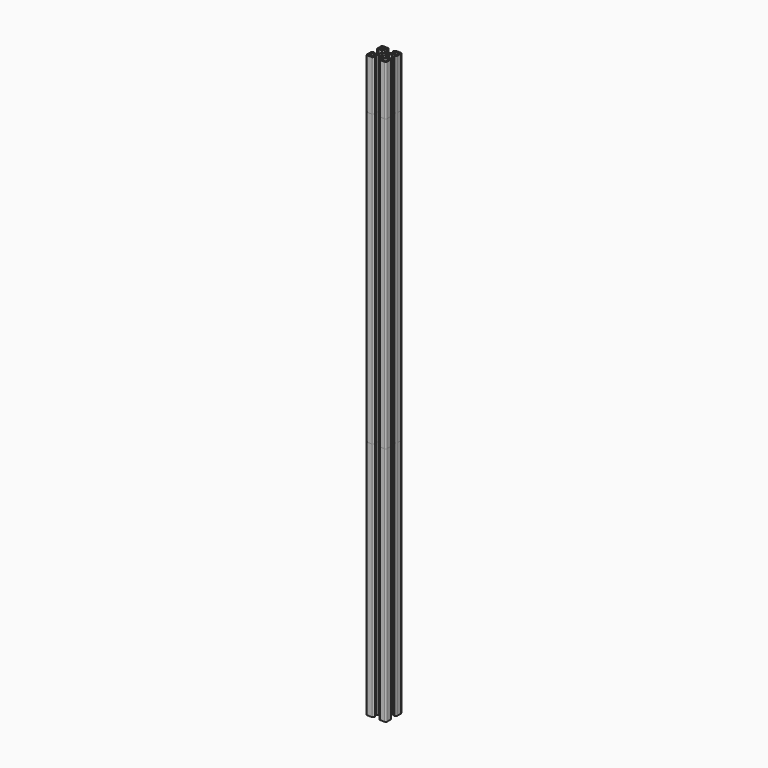
from build123d import *

# Parameters (mm, degrees)
F0_R     = 2.1
F1_DEPTH = 340
F2_DEPTH = 240
F3_DEPTH = 290


# Not quite as in the source:
# - ends of sketch curves that miss each other by under 0.0002 mm in the source are joined


with BuildPart() as f1:
    # F0 (on Top) → F1 (new body)
    with BuildSketch(Plane.XY):
        with BuildLine():
            ThreePointArc((-9.7686134352, -3.6910416547), (-9.9398646382, -3.9473364469), (-10.0000000781, -4.2496570118))
            Line((-10.0000000781, -4.2496570118), (-10.0000000781, -8.5808970118))
            ThreePointArc((-10.0000000781, -8.5808970118), (-9.5692783777, -9.55712574), (-8.5985020649, -9.9999998067))
            Line((-8.5985020649, -9.9999998067), (-4.0428310781, -10.0000000118))
            ThreePointArc((-4.0428310781, -10.0000000118), (-3.7366840055, -9.9391035025), (-3.4771451531, -9.7656849367))
            Line((-3.4771451531, -9.7656849367), (-2.3732230781, -8.6617630118))
            ThreePointArc((-2.3732230781, -8.6617630118), (-2.3190301949, -8.3893151537), (-2.5500000781, -8.2349860118))
            Line((-2.5500000781, -8.2349860118), (-3.6000000781, -8.2349860118))
            Line((-3.6000000781, -8.2349860118), (-3.6000000781, -5.0349860118))
            Line((-3.6000000781, -5.0349860118), (-2.0054060781, -3.4349860118))
            Line((-2.0054060781, -3.4349860118), (-0.3000000781, -3.4349860118))
            Line((-0.3000000781, -3.4349860118), (-7.81e-08, -3.1750330118))
            Line((-7.81e-08, -3.1750330118), (0.2999999219, -3.4349860118))
            Line((0.2999999219, -3.4349860118), (2.0054059219, -3.4349860118))
            Line((2.0054059219, -3.4349860118), (3.5999999219, -5.0349860118))
            Line((3.5999999219, -5.0349860118), (3.5999999219, -8.2349860118))
            Line((3.5999999219, -8.2349860118), (2.5499999219, -8.2349860118))
            ThreePointArc((2.5499999219, -8.2349860118), (2.3190299035, -8.3893154803), (2.3732237266, -8.6617632071))
            Line((2.3732237266, -8.6617632071), (3.4771459219, -9.7656850118))
            ThreePointArc((3.4771459219, -9.7656850118), (3.736684176, -9.9391036378), (4.0428309219, -10.0000000118))
            Line((4.0428309219, -10.0000000118), (8.5985019219, -10.0000000118))
            ThreePointArc((8.5985019219, -10.0000000118), (9.5692782397, -9.5571257216), (10.0000004186, -8.5808969857))
            Line((10.0000004186, -8.5808969857), (9.9999999219, -4.2496570118))
            ThreePointArc((9.9999999219, -4.2496570118), (9.9398646173, -3.9473367736), (9.7686137791, -3.6910421547))
            Line((9.7686137791, -3.6910421547), (8.4861509219, -2.4085790118))
            ThreePointArc((8.4861509219, -2.4085790118), (8.2729345349, -2.363330341), (8.1449896008, -2.5397919954))
            Line((8.1449896008, -2.5397919954), (8.1449899219, -3.6000000118))
            Line((8.1449899219, -3.6000000118), (5.0283829219, -3.6000000118))
            Line((5.0283829219, -3.6000000118), (3.3999999219, -1.9660960118))
            Line((3.3999999219, -1.9660960118), (3.3999999219, -0.3808970118))
            Line((3.3999999219, -0.3808970118), (3.0191029219, -1.18e-08))
            Line((3.0191029219, -1.18e-08), (3.3999999219, 0.3808969882))
            Line((3.3999999219, 0.3808969882), (3.3999999219, 1.9660959882))
            Line((3.3999999219, 1.9660959882), (5.0283829219, 3.5999999882))
            Line((5.0283829219, 3.5999999882), (8.1449899219, 3.5999999882))
            Line((8.1449899219, 3.5999999882), (8.1449899219, 2.5397919882))
            ThreePointArc((8.1449899219, 2.5397919882), (8.2729345349, 2.3633303174), (8.4861507782, 2.408579132))
            Line((8.4861507782, 2.408579132), (9.7686139219, 3.6910419882))
            ThreePointArc((9.7686139219, 3.6910419882), (9.9398646173, 3.94733675), (9.9999999219, 4.2496569882))
            Line((9.9999999219, 4.2496569882), (9.9999999219, 8.5808969882))
            ThreePointArc((9.9999999219, 8.5808969882), (9.5692782397, 9.557125698), (8.5985019087, 9.9999997831))
            Line((8.5985019087, 9.9999997831), (4.0428309219, 9.9999999882))
            ThreePointArc((4.0428309219, 9.9999999882), (3.7366845027, 9.9391037495), (3.477145997, 9.7656859132))
            Line((3.477145997, 9.7656859132), (2.3732229219, 8.6617629882))
            ThreePointArc((2.3732229219, 8.6617629882), (2.3190299035, 8.3893154568), (2.5499999219, 8.2349859882))
            Line((2.5499999219, 8.2349859882), (3.5999999219, 8.2349859882))
            Line((3.5999999219, 8.2349859882), (3.5999999219, 5.0349859882))
            Line((3.5999999219, 5.0349859882), (2.0054059219, 3.4349859882))
            Line((2.0054059219, 3.4349859882), (0.2999999219, 3.4349859882))
            Line((0.2999999219, 3.4349859882), (-7.81e-08, 3.1750329882))
            Line((-7.81e-08, 3.1750329882), (-0.3000000781, 3.4349859882))
            Line((-0.3000000781, 3.4349859882), (-2.0054060781, 3.4349859882))
            Line((-2.0054060781, 3.4349859882), (-3.6000000781, 5.0349859882))
            Line((-3.6000000781, 5.0349859882), (-3.6000000781, 8.2349859882))
            Line((-3.6000000781, 8.2349859882), (-2.5500000781, 8.2349859882))
            ThreePointArc((-2.5500000781, 8.2349859882), (-2.3190301949, 8.3893151301), (-2.3732233828, 8.6617626835))
            Line((-2.3732233828, 8.6617626835), (-3.4771460781, 9.7656849882))
            ThreePointArc((-3.4771460781, 9.7656849882), (-3.7366843322, 9.9391036142), (-4.0428310781, 9.9999999882))
            Line((-4.0428310781, 9.9999999882), (-8.5985020781, 9.9999999882))
            ThreePointArc((-8.5985020781, 9.9999999882), (-9.5692783777, 9.5571257164), (-10.0000005721, 8.5808970139))
            Line((-10.0000005721, 8.5808970139), (-10.0000000781, 4.2496569882))
            ThreePointArc((-10.0000000781, 4.2496569882), (-9.9398646382, 3.9473364234), (-9.7686134352, 3.6910416311))
            Line((-9.7686134352, 3.6910416311), (-8.4861510781, 2.4085789882))
            ThreePointArc((-8.4861510781, 2.4085789882), (-8.2729343372, 2.3633304535), (-8.1449897544, 2.5397920228))
            Line((-8.1449897544, 2.5397920228), (-8.1449900781, 3.5999999882))
            Line((-8.1449900781, 3.5999999882), (-5.0283830781, 3.5999999882))
            Line((-5.0283830781, 3.5999999882), (-3.4000000781, 1.9660959882))
            Line((-3.4000000781, 1.9660959882), (-3.4000000781, 0.3808969882))
            Line((-3.4000000781, 0.3808969882), (-3.0191030781, -1.18e-08))
            Line((-3.0191030781, -1.18e-08), (-3.4000000781, -0.3808970118))
            Line((-3.4000000781, -0.3808970118), (-3.4000000781, -1.9660960118))
            Line((-3.4000000781, -1.9660960118), (-5.0283830781, -3.6000000118))
            Line((-5.0283830781, -3.6000000118), (-8.1449900781, -3.6000000118))
            Line((-8.1449900781, -3.6000000118), (-8.1449900781, -2.5397920118))
            ThreePointArc((-8.1449900781, -2.5397920118), (-8.2729343372, -2.3633304771), (-8.4861504343, -2.4085786556))
            Line((-8.4861504343, -2.4085786556), (-9.7686134352, -3.6910416547))
        make_face()
        with BuildLine():
            Line((-8.3887380781, -4.8000000118), (-5.3887380781, -4.8000000118))
            ThreePointArc((-5.3887380781, -4.8000000118), (-4.9405858182, -4.9345893802), (-4.7999996469, -5.3808969072))
            Line((-4.7999996469, -5.3808969072), (-4.8000000781, -8.3808970118))
            ThreePointArc((-4.8000000781, -8.3808970118), (-5.0082631765, -8.7203831526), (-5.3985012393, -8.7999997745))
            Line((-5.3985012393, -8.7999997745), (-8.3985020781, -8.8000000118))
            ThreePointArc((-8.3985020781, -8.8000000118), (-8.6662843252, -8.6546658791), (-8.8000004374, -8.3808970642))
            Line((-8.8000004374, -8.3808970642), (-8.8000000781, -5.3808970118))
            ThreePointArc((-8.8000000781, -5.3808970118), (-8.7157976891, -5.0044798887), (-8.3887380781, -4.8000000118))
        make_face(mode=Mode.SUBTRACT)
        with Locations((-7.81e-08, -1.18e-08)):
            Circle(F0_R, mode=Mode.SUBTRACT)
        with BuildLine():
            ThreePointArc((8.3887379109, -4.800000079), (8.7157974824, -5.0044798173), (8.8000002705, -5.380896896))
            Line((8.8000002705, -5.380896896), (8.8000009219, -8.3808970118))
            ThreePointArc((8.8000009219, -8.3808970118), (8.6662842189, -8.654665827), (8.3985019428, -8.8000001216))
            Line((8.3985019428, -8.8000001216), (5.3985019219, -8.8000000118))
            ThreePointArc((5.3985019219, -8.8000000118), (5.0082634784, -8.7203834734), (4.7999996354, -8.3808970523))
            Line((4.7999996354, -8.3808970523), (4.7999999219, -5.3808970118))
            ThreePointArc((4.7999999219, -5.3808970118), (4.9405855977, -4.9345894436), (5.3887379814, -4.7999997112))
            Line((5.3887379814, -4.7999997112), (8.3887379109, -4.800000079))
        make_face(mode=Mode.SUBTRACT)
        with BuildLine():
            ThreePointArc((-8.388738067, 4.8000000554), (-8.7157976891, 5.0044798651), (-8.800000396, 5.3808970447))
            Line((-8.800000396, 5.3808970447), (-8.8000000781, 8.3808969882))
            ThreePointArc((-8.8000000781, 8.3808969882), (-8.6662843252, 8.6546658555), (-8.3985020989, 8.800000098))
            Line((-8.3985020989, 8.800000098), (-5.3985020781, 8.7999999882))
            ThreePointArc((-5.3985020781, 8.7999999882), (-5.0082630918, 8.7203830697), (-4.7999997719, 8.38089689))
            Line((-4.7999997719, 8.38089689), (-4.8000000781, 5.3808969882))
            ThreePointArc((-4.8000000781, 5.3808969882), (-4.9405858182, 4.9345893566), (-5.3887381375, 4.7999996876))
            Line((-5.3887381375, 4.7999996876), (-8.388738067, 4.8000000554))
        make_face(mode=Mode.SUBTRACT)
        with BuildLine():
            Line((8.3887379219, 4.7999999882), (5.3887379219, 4.7999999882))
            ThreePointArc((5.3887379219, 4.7999999882), (4.9405855977, 4.9345894201), (4.7999995234, 5.3808970615))
            Line((4.7999995234, 5.3808970615), (4.7999999219, 8.3808969882))
            ThreePointArc((4.7999999219, 8.3808969882), (5.0082633937, 8.7203833905), (5.398501838, 8.7999995913))
            Line((5.398501838, 8.7999995913), (8.3985019219, 8.7999999882))
            ThreePointArc((8.3985019219, 8.7999999882), (8.6662842189, 8.6546658035), (8.8000003021, 8.3808968979))
            Line((8.8000003021, 8.3808968979), (8.7999999219, 5.3808969882))
            ThreePointArc((8.7999999219, 5.3808969882), (8.7157974824, 5.0044797937), (8.3887379219, 4.7999999882))
        make_face(mode=Mode.SUBTRACT)
    extrude(amount=F1_DEPTH)


with BuildPart() as f2:
    # F0 (on Top) → F2 (new body)
    with BuildSketch(Plane.XY):
        with BuildLine():
            ThreePointArc((-9.7686134352, -3.6910416547), (-9.9398646382, -3.9473364469), (-10.0000000781, -4.2496570118))
            Line((-10.0000000781, -4.2496570118), (-10.0000000781, -8.5808970118))
            ThreePointArc((-10.0000000781, -8.5808970118), (-9.5692783777, -9.55712574), (-8.5985020649, -9.9999998067))
            Line((-8.5985020649, -9.9999998067), (-4.0428310781, -10.0000000118))
            ThreePointArc((-4.0428310781, -10.0000000118), (-3.7366840055, -9.9391035025), (-3.4771451531, -9.7656849367))
            Line((-3.4771451531, -9.7656849367), (-2.3732230781, -8.6617630118))
            ThreePointArc((-2.3732230781, -8.6617630118), (-2.3190301949, -8.3893151537), (-2.5500000781, -8.2349860118))
            Line((-2.5500000781, -8.2349860118), (-3.6000000781, -8.2349860118))
            Line((-3.6000000781, -8.2349860118), (-3.6000000781, -5.0349860118))
            Line((-3.6000000781, -5.0349860118), (-2.0054060781, -3.4349860118))
            Line((-2.0054060781, -3.4349860118), (-0.3000000781, -3.4349860118))
            Line((-0.3000000781, -3.4349860118), (-7.81e-08, -3.1750330118))
            Line((-7.81e-08, -3.1750330118), (0.2999999219, -3.4349860118))
            Line((0.2999999219, -3.4349860118), (2.0054059219, -3.4349860118))
            Line((2.0054059219, -3.4349860118), (3.5999999219, -5.0349860118))
            Line((3.5999999219, -5.0349860118), (3.5999999219, -8.2349860118))
            Line((3.5999999219, -8.2349860118), (2.5499999219, -8.2349860118))
            ThreePointArc((2.5499999219, -8.2349860118), (2.3190299035, -8.3893154803), (2.3732237266, -8.6617632071))
            Line((2.3732237266, -8.6617632071), (3.4771459219, -9.7656850118))
            ThreePointArc((3.4771459219, -9.7656850118), (3.736684176, -9.9391036378), (4.0428309219, -10.0000000118))
            Line((4.0428309219, -10.0000000118), (8.5985019219, -10.0000000118))
            ThreePointArc((8.5985019219, -10.0000000118), (9.5692782397, -9.5571257216), (10.0000004186, -8.5808969857))
            Line((10.0000004186, -8.5808969857), (9.9999999219, -4.2496570118))
            ThreePointArc((9.9999999219, -4.2496570118), (9.9398646173, -3.9473367736), (9.7686137791, -3.6910421547))
            Line((9.7686137791, -3.6910421547), (8.4861509219, -2.4085790118))
            ThreePointArc((8.4861509219, -2.4085790118), (8.2729345349, -2.363330341), (8.1449896008, -2.5397919954))
            Line((8.1449896008, -2.5397919954), (8.1449899219, -3.6000000118))
            Line((8.1449899219, -3.6000000118), (5.0283829219, -3.6000000118))
            Line((5.0283829219, -3.6000000118), (3.3999999219, -1.9660960118))
            Line((3.3999999219, -1.9660960118), (3.3999999219, -0.3808970118))
            Line((3.3999999219, -0.3808970118), (3.0191029219, -1.18e-08))
            Line((3.0191029219, -1.18e-08), (3.3999999219, 0.3808969882))
            Line((3.3999999219, 0.3808969882), (3.3999999219, 1.9660959882))
            Line((3.3999999219, 1.9660959882), (5.0283829219, 3.5999999882))
            Line((5.0283829219, 3.5999999882), (8.1449899219, 3.5999999882))
            Line((8.1449899219, 3.5999999882), (8.1449899219, 2.5397919882))
            ThreePointArc((8.1449899219, 2.5397919882), (8.2729345349, 2.3633303174), (8.4861507782, 2.408579132))
            Line((8.4861507782, 2.408579132), (9.7686139219, 3.6910419882))
            ThreePointArc((9.7686139219, 3.6910419882), (9.9398646173, 3.94733675), (9.9999999219, 4.2496569882))
            Line((9.9999999219, 4.2496569882), (9.9999999219, 8.5808969882))
            ThreePointArc((9.9999999219, 8.5808969882), (9.5692782397, 9.557125698), (8.5985019087, 9.9999997831))
            Line((8.5985019087, 9.9999997831), (4.0428309219, 9.9999999882))
            ThreePointArc((4.0428309219, 9.9999999882), (3.7366845027, 9.9391037495), (3.477145997, 9.7656859132))
            Line((3.477145997, 9.7656859132), (2.3732229219, 8.6617629882))
            ThreePointArc((2.3732229219, 8.6617629882), (2.3190299035, 8.3893154568), (2.5499999219, 8.2349859882))
            Line((2.5499999219, 8.2349859882), (3.5999999219, 8.2349859882))
            Line((3.5999999219, 8.2349859882), (3.5999999219, 5.0349859882))
            Line((3.5999999219, 5.0349859882), (2.0054059219, 3.4349859882))
            Line((2.0054059219, 3.4349859882), (0.2999999219, 3.4349859882))
            Line((0.2999999219, 3.4349859882), (-7.81e-08, 3.1750329882))
            Line((-7.81e-08, 3.1750329882), (-0.3000000781, 3.4349859882))
            Line((-0.3000000781, 3.4349859882), (-2.0054060781, 3.4349859882))
            Line((-2.0054060781, 3.4349859882), (-3.6000000781, 5.0349859882))
            Line((-3.6000000781, 5.0349859882), (-3.6000000781, 8.2349859882))
            Line((-3.6000000781, 8.2349859882), (-2.5500000781, 8.2349859882))
            ThreePointArc((-2.5500000781, 8.2349859882), (-2.3190301949, 8.3893151301), (-2.3732233828, 8.6617626835))
            Line((-2.3732233828, 8.6617626835), (-3.4771460781, 9.7656849882))
            ThreePointArc((-3.4771460781, 9.7656849882), (-3.7366843322, 9.9391036142), (-4.0428310781, 9.9999999882))
            Line((-4.0428310781, 9.9999999882), (-8.5985020781, 9.9999999882))
            ThreePointArc((-8.5985020781, 9.9999999882), (-9.5692783777, 9.5571257164), (-10.0000005721, 8.5808970139))
            Line((-10.0000005721, 8.5808970139), (-10.0000000781, 4.2496569882))
            ThreePointArc((-10.0000000781, 4.2496569882), (-9.9398646382, 3.9473364234), (-9.7686134352, 3.6910416311))
            Line((-9.7686134352, 3.6910416311), (-8.4861510781, 2.4085789882))
            ThreePointArc((-8.4861510781, 2.4085789882), (-8.2729343372, 2.3633304535), (-8.1449897544, 2.5397920228))
            Line((-8.1449897544, 2.5397920228), (-8.1449900781, 3.5999999882))
            Line((-8.1449900781, 3.5999999882), (-5.0283830781, 3.5999999882))
            Line((-5.0283830781, 3.5999999882), (-3.4000000781, 1.9660959882))
            Line((-3.4000000781, 1.9660959882), (-3.4000000781, 0.3808969882))
            Line((-3.4000000781, 0.3808969882), (-3.0191030781, -1.18e-08))
            Line((-3.0191030781, -1.18e-08), (-3.4000000781, -0.3808970118))
            Line((-3.4000000781, -0.3808970118), (-3.4000000781, -1.9660960118))
            Line((-3.4000000781, -1.9660960118), (-5.0283830781, -3.6000000118))
            Line((-5.0283830781, -3.6000000118), (-8.1449900781, -3.6000000118))
            Line((-8.1449900781, -3.6000000118), (-8.1449900781, -2.5397920118))
            ThreePointArc((-8.1449900781, -2.5397920118), (-8.2729343372, -2.3633304771), (-8.4861504343, -2.4085786556))
            Line((-8.4861504343, -2.4085786556), (-9.7686134352, -3.6910416547))
        make_face()
        with BuildLine():
            Line((-8.3887380781, -4.8000000118), (-5.3887380781, -4.8000000118))
            ThreePointArc((-5.3887380781, -4.8000000118), (-4.9405858182, -4.9345893802), (-4.7999996469, -5.3808969072))
            Line((-4.7999996469, -5.3808969072), (-4.8000000781, -8.3808970118))
            ThreePointArc((-4.8000000781, -8.3808970118), (-5.0082631765, -8.7203831526), (-5.3985012393, -8.7999997745))
            Line((-5.3985012393, -8.7999997745), (-8.3985020781, -8.8000000118))
            ThreePointArc((-8.3985020781, -8.8000000118), (-8.6662843252, -8.6546658791), (-8.8000004374, -8.3808970642))
            Line((-8.8000004374, -8.3808970642), (-8.8000000781, -5.3808970118))
            ThreePointArc((-8.8000000781, -5.3808970118), (-8.7157976891, -5.0044798887), (-8.3887380781, -4.8000000118))
        make_face(mode=Mode.SUBTRACT)
        with Locations((-7.81e-08, -1.18e-08)):
            Circle(F0_R, mode=Mode.SUBTRACT)
        with BuildLine():
            ThreePointArc((8.3887379109, -4.800000079), (8.7157974824, -5.0044798173), (8.8000002705, -5.380896896))
            Line((8.8000002705, -5.380896896), (8.8000009219, -8.3808970118))
            ThreePointArc((8.8000009219, -8.3808970118), (8.6662842189, -8.654665827), (8.3985019428, -8.8000001216))
            Line((8.3985019428, -8.8000001216), (5.3985019219, -8.8000000118))
            ThreePointArc((5.3985019219, -8.8000000118), (5.0082634784, -8.7203834734), (4.7999996354, -8.3808970523))
            Line((4.7999996354, -8.3808970523), (4.7999999219, -5.3808970118))
            ThreePointArc((4.7999999219, -5.3808970118), (4.9405855977, -4.9345894436), (5.3887379814, -4.7999997112))
            Line((5.3887379814, -4.7999997112), (8.3887379109, -4.800000079))
        make_face(mode=Mode.SUBTRACT)
        with BuildLine():
            ThreePointArc((-8.388738067, 4.8000000554), (-8.7157976891, 5.0044798651), (-8.800000396, 5.3808970447))
            Line((-8.800000396, 5.3808970447), (-8.8000000781, 8.3808969882))
            ThreePointArc((-8.8000000781, 8.3808969882), (-8.6662843252, 8.6546658555), (-8.3985020989, 8.800000098))
            Line((-8.3985020989, 8.800000098), (-5.3985020781, 8.7999999882))
            ThreePointArc((-5.3985020781, 8.7999999882), (-5.0082630918, 8.7203830697), (-4.7999997719, 8.38089689))
            Line((-4.7999997719, 8.38089689), (-4.8000000781, 5.3808969882))
            ThreePointArc((-4.8000000781, 5.3808969882), (-4.9405858182, 4.9345893566), (-5.3887381375, 4.7999996876))
            Line((-5.3887381375, 4.7999996876), (-8.388738067, 4.8000000554))
        make_face(mode=Mode.SUBTRACT)
        with BuildLine():
            Line((8.3887379219, 4.7999999882), (5.3887379219, 4.7999999882))
            ThreePointArc((5.3887379219, 4.7999999882), (4.9405855977, 4.9345894201), (4.7999995234, 5.3808970615))
            Line((4.7999995234, 5.3808970615), (4.7999999219, 8.3808969882))
            ThreePointArc((4.7999999219, 8.3808969882), (5.0082633937, 8.7203833905), (5.398501838, 8.7999995913))
            Line((5.398501838, 8.7999995913), (8.3985019219, 8.7999999882))
            ThreePointArc((8.3985019219, 8.7999999882), (8.6662842189, 8.6546658035), (8.8000003021, 8.3808968979))
            Line((8.8000003021, 8.3808968979), (8.7999999219, 5.3808969882))
            ThreePointArc((8.7999999219, 5.3808969882), (8.7157974824, 5.0044797937), (8.3887379219, 4.7999999882))
        make_face(mode=Mode.SUBTRACT)
    extrude(amount=-F2_DEPTH)


with BuildPart() as f3:
    # F0 (on Top) → F3 (new body)
    with BuildSketch(Plane.XY):
        with BuildLine():
            ThreePointArc((-9.7686134352, -3.6910416547), (-9.9398646382, -3.9473364469), (-10.0000000781, -4.2496570118))
            Line((-10.0000000781, -4.2496570118), (-10.0000000781, -8.5808970118))
            ThreePointArc((-10.0000000781, -8.5808970118), (-9.5692783777, -9.55712574), (-8.5985020649, -9.9999998067))
            Line((-8.5985020649, -9.9999998067), (-4.0428310781, -10.0000000118))
            ThreePointArc((-4.0428310781, -10.0000000118), (-3.7366840055, -9.9391035025), (-3.4771451531, -9.7656849367))
            Line((-3.4771451531, -9.7656849367), (-2.3732230781, -8.6617630118))
            ThreePointArc((-2.3732230781, -8.6617630118), (-2.3190301949, -8.3893151537), (-2.5500000781, -8.2349860118))
            Line((-2.5500000781, -8.2349860118), (-3.6000000781, -8.2349860118))
            Line((-3.6000000781, -8.2349860118), (-3.6000000781, -5.0349860118))
            Line((-3.6000000781, -5.0349860118), (-2.0054060781, -3.4349860118))
            Line((-2.0054060781, -3.4349860118), (-0.3000000781, -3.4349860118))
            Line((-0.3000000781, -3.4349860118), (-7.81e-08, -3.1750330118))
            Line((-7.81e-08, -3.1750330118), (0.2999999219, -3.4349860118))
            Line((0.2999999219, -3.4349860118), (2.0054059219, -3.4349860118))
            Line((2.0054059219, -3.4349860118), (3.5999999219, -5.0349860118))
            Line((3.5999999219, -5.0349860118), (3.5999999219, -8.2349860118))
            Line((3.5999999219, -8.2349860118), (2.5499999219, -8.2349860118))
            ThreePointArc((2.5499999219, -8.2349860118), (2.3190299035, -8.3893154803), (2.3732237266, -8.6617632071))
            Line((2.3732237266, -8.6617632071), (3.4771459219, -9.7656850118))
            ThreePointArc((3.4771459219, -9.7656850118), (3.736684176, -9.9391036378), (4.0428309219, -10.0000000118))
            Line((4.0428309219, -10.0000000118), (8.5985019219, -10.0000000118))
            ThreePointArc((8.5985019219, -10.0000000118), (9.5692782397, -9.5571257216), (10.0000004186, -8.5808969857))
            Line((10.0000004186, -8.5808969857), (9.9999999219, -4.2496570118))
            ThreePointArc((9.9999999219, -4.2496570118), (9.9398646173, -3.9473367736), (9.7686137791, -3.6910421547))
            Line((9.7686137791, -3.6910421547), (8.4861509219, -2.4085790118))
            ThreePointArc((8.4861509219, -2.4085790118), (8.2729345349, -2.363330341), (8.1449896008, -2.5397919954))
            Line((8.1449896008, -2.5397919954), (8.1449899219, -3.6000000118))
            Line((8.1449899219, -3.6000000118), (5.0283829219, -3.6000000118))
            Line((5.0283829219, -3.6000000118), (3.3999999219, -1.9660960118))
            Line((3.3999999219, -1.9660960118), (3.3999999219, -0.3808970118))
            Line((3.3999999219, -0.3808970118), (3.0191029219, -1.18e-08))
            Line((3.0191029219, -1.18e-08), (3.3999999219, 0.3808969882))
            Line((3.3999999219, 0.3808969882), (3.3999999219, 1.9660959882))
            Line((3.3999999219, 1.9660959882), (5.0283829219, 3.5999999882))
            Line((5.0283829219, 3.5999999882), (8.1449899219, 3.5999999882))
            Line((8.1449899219, 3.5999999882), (8.1449899219, 2.5397919882))
            ThreePointArc((8.1449899219, 2.5397919882), (8.2729345349, 2.3633303174), (8.4861507782, 2.408579132))
            Line((8.4861507782, 2.408579132), (9.7686139219, 3.6910419882))
            ThreePointArc((9.7686139219, 3.6910419882), (9.9398646173, 3.94733675), (9.9999999219, 4.2496569882))
            Line((9.9999999219, 4.2496569882), (9.9999999219, 8.5808969882))
            ThreePointArc((9.9999999219, 8.5808969882), (9.5692782397, 9.557125698), (8.5985019087, 9.9999997831))
            Line((8.5985019087, 9.9999997831), (4.0428309219, 9.9999999882))
            ThreePointArc((4.0428309219, 9.9999999882), (3.7366845027, 9.9391037495), (3.477145997, 9.7656859132))
            Line((3.477145997, 9.7656859132), (2.3732229219, 8.6617629882))
            ThreePointArc((2.3732229219, 8.6617629882), (2.3190299035, 8.3893154568), (2.5499999219, 8.2349859882))
            Line((2.5499999219, 8.2349859882), (3.5999999219, 8.2349859882))
            Line((3.5999999219, 8.2349859882), (3.5999999219, 5.0349859882))
            Line((3.5999999219, 5.0349859882), (2.0054059219, 3.4349859882))
            Line((2.0054059219, 3.4349859882), (0.2999999219, 3.4349859882))
            Line((0.2999999219, 3.4349859882), (-7.81e-08, 3.1750329882))
            Line((-7.81e-08, 3.1750329882), (-0.3000000781, 3.4349859882))
            Line((-0.3000000781, 3.4349859882), (-2.0054060781, 3.4349859882))
            Line((-2.0054060781, 3.4349859882), (-3.6000000781, 5.0349859882))
            Line((-3.6000000781, 5.0349859882), (-3.6000000781, 8.2349859882))
            Line((-3.6000000781, 8.2349859882), (-2.5500000781, 8.2349859882))
            ThreePointArc((-2.5500000781, 8.2349859882), (-2.3190301949, 8.3893151301), (-2.3732233828, 8.6617626835))
            Line((-2.3732233828, 8.6617626835), (-3.4771460781, 9.7656849882))
            ThreePointArc((-3.4771460781, 9.7656849882), (-3.7366843322, 9.9391036142), (-4.0428310781, 9.9999999882))
            Line((-4.0428310781, 9.9999999882), (-8.5985020781, 9.9999999882))
            ThreePointArc((-8.5985020781, 9.9999999882), (-9.5692783777, 9.5571257164), (-10.0000005721, 8.5808970139))
            Line((-10.0000005721, 8.5808970139), (-10.0000000781, 4.2496569882))
            ThreePointArc((-10.0000000781, 4.2496569882), (-9.9398646382, 3.9473364234), (-9.7686134352, 3.6910416311))
            Line((-9.7686134352, 3.6910416311), (-8.4861510781, 2.4085789882))
            ThreePointArc((-8.4861510781, 2.4085789882), (-8.2729343372, 2.3633304535), (-8.1449897544, 2.5397920228))
            Line((-8.1449897544, 2.5397920228), (-8.1449900781, 3.5999999882))
            Line((-8.1449900781, 3.5999999882), (-5.0283830781, 3.5999999882))
            Line((-5.0283830781, 3.5999999882), (-3.4000000781, 1.9660959882))
            Line((-3.4000000781, 1.9660959882), (-3.4000000781, 0.3808969882))
            Line((-3.4000000781, 0.3808969882), (-3.0191030781, -1.18e-08))
            Line((-3.0191030781, -1.18e-08), (-3.4000000781, -0.3808970118))
            Line((-3.4000000781, -0.3808970118), (-3.4000000781, -1.9660960118))
            Line((-3.4000000781, -1.9660960118), (-5.0283830781, -3.6000000118))
            Line((-5.0283830781, -3.6000000118), (-8.1449900781, -3.6000000118))
            Line((-8.1449900781, -3.6000000118), (-8.1449900781, -2.5397920118))
            ThreePointArc((-8.1449900781, -2.5397920118), (-8.2729343372, -2.3633304771), (-8.4861504343, -2.4085786556))
            Line((-8.4861504343, -2.4085786556), (-9.7686134352, -3.6910416547))
        make_face()
        with BuildLine():
            Line((-8.3887380781, -4.8000000118), (-5.3887380781, -4.8000000118))
            ThreePointArc((-5.3887380781, -4.8000000118), (-4.9405858182, -4.9345893802), (-4.7999996469, -5.3808969072))
            Line((-4.7999996469, -5.3808969072), (-4.8000000781, -8.3808970118))
            ThreePointArc((-4.8000000781, -8.3808970118), (-5.0082631765, -8.7203831526), (-5.3985012393, -8.7999997745))
            Line((-5.3985012393, -8.7999997745), (-8.3985020781, -8.8000000118))
            ThreePointArc((-8.3985020781, -8.8000000118), (-8.6662843252, -8.6546658791), (-8.8000004374, -8.3808970642))
            Line((-8.8000004374, -8.3808970642), (-8.8000000781, -5.3808970118))
            ThreePointArc((-8.8000000781, -5.3808970118), (-8.7157976891, -5.0044798887), (-8.3887380781, -4.8000000118))
        make_face(mode=Mode.SUBTRACT)
        with Locations((-7.81e-08, -1.18e-08)):
            Circle(F0_R, mode=Mode.SUBTRACT)
        with BuildLine():
            ThreePointArc((8.3887379109, -4.800000079), (8.7157974824, -5.0044798173), (8.8000002705, -5.380896896))
            Line((8.8000002705, -5.380896896), (8.8000009219, -8.3808970118))
            ThreePointArc((8.8000009219, -8.3808970118), (8.6662842189, -8.654665827), (8.3985019428, -8.8000001216))
            Line((8.3985019428, -8.8000001216), (5.3985019219, -8.8000000118))
            ThreePointArc((5.3985019219, -8.8000000118), (5.0082634784, -8.7203834734), (4.7999996354, -8.3808970523))
            Line((4.7999996354, -8.3808970523), (4.7999999219, -5.3808970118))
            ThreePointArc((4.7999999219, -5.3808970118), (4.9405855977, -4.9345894436), (5.3887379814, -4.7999997112))
            Line((5.3887379814, -4.7999997112), (8.3887379109, -4.800000079))
        make_face(mode=Mode.SUBTRACT)
        with BuildLine():
            ThreePointArc((-8.388738067, 4.8000000554), (-8.7157976891, 5.0044798651), (-8.800000396, 5.3808970447))
            Line((-8.800000396, 5.3808970447), (-8.8000000781, 8.3808969882))
            ThreePointArc((-8.8000000781, 8.3808969882), (-8.6662843252, 8.6546658555), (-8.3985020989, 8.800000098))
            Line((-8.3985020989, 8.800000098), (-5.3985020781, 8.7999999882))
            ThreePointArc((-5.3985020781, 8.7999999882), (-5.0082630918, 8.7203830697), (-4.7999997719, 8.38089689))
            Line((-4.7999997719, 8.38089689), (-4.8000000781, 5.3808969882))
            ThreePointArc((-4.8000000781, 5.3808969882), (-4.9405858182, 4.9345893566), (-5.3887381375, 4.7999996876))
            Line((-5.3887381375, 4.7999996876), (-8.388738067, 4.8000000554))
        make_face(mode=Mode.SUBTRACT)
        with BuildLine():
            Line((8.3887379219, 4.7999999882), (5.3887379219, 4.7999999882))
            ThreePointArc((5.3887379219, 4.7999999882), (4.9405855977, 4.9345894201), (4.7999995234, 5.3808970615))
            Line((4.7999995234, 5.3808970615), (4.7999999219, 8.3808969882))
            ThreePointArc((4.7999999219, 8.3808969882), (5.0082633937, 8.7203833905), (5.398501838, 8.7999995913))
            Line((5.398501838, 8.7999995913), (8.3985019219, 8.7999999882))
            ThreePointArc((8.3985019219, 8.7999999882), (8.6662842189, 8.6546658035), (8.8000003021, 8.3808968979))
            Line((8.8000003021, 8.3808968979), (8.7999999219, 5.3808969882))
            ThreePointArc((8.7999999219, 5.3808969882), (8.7157974824, 5.0044797937), (8.3887379219, 4.7999999882))
        make_face(mode=Mode.SUBTRACT)
    extrude(amount=F3_DEPTH)


solid = Compound([f1.part, f2.part, f3.part])
